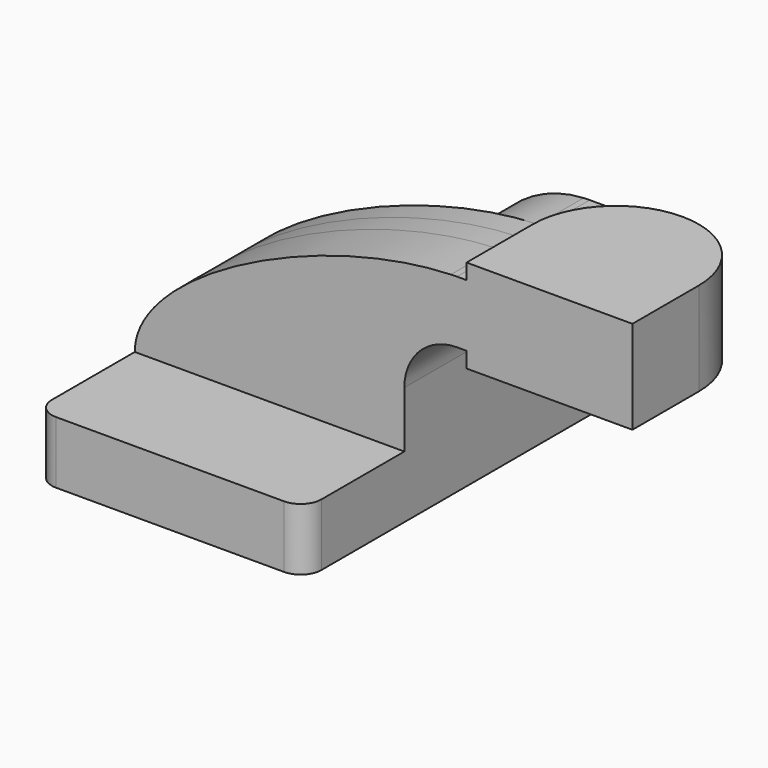
from build123d import *

# Parameters (mm, degrees)
F1_DEPTH = 63.5
F0_W     = 25.4
F0_H     = 19.05
F2_DEPTH = 25.4
F3_DEPTH = 7.9375
F5_R     = 6.35
F0_H_2   = 4.7752
F0_H_3   = 4.7498
F6_DEPTH = 25.4


with BuildPart() as f1:
    # F0 (on Front) → F1 (new body, symmetric)
    with BuildSketch(Plane.XZ):
        Polygon((-41.275, -9.525), (41.275, -9.525), (41.275, 9.525), (22.225, 9.525), (-41.275, 9.525), align=None)
    extrude(amount=F1_DEPTH, both=True)

    # F0 (on Front) → F2 (join, symmetric)
    with BuildSketch(Plane.XZ):
        with BuildLine():
            Line((22.225, 9.525), (41.275, 9.525))
            Line((41.275, 9.525), (41.275, 26.7462))
            ThreePointArc((41.275, 26.7462), (45.9990747262, 38.1511252738), (57.404, 42.8752))
            Line((57.404, 42.8752), (60.325, 42.8752))
            Line((60.325, 42.8752), (60.325, 61.9252))
            Line((60.325, 61.9252), (57.404, 61.9252))
            add(Edge.make_bspline(
                [(55.5422575952, 61.875901909), (56.1662788609, 61.89841175), (56.7869415526, 61.914880349), (57.404, 61.9252)],
                knots=[110.0591294768, 110.0591294768, 110.0591294768, 110.0591294768, 111.7288056011, 111.7288056011, 111.7288056011, 111.7288056011], degree=3))
            ThreePointArc((55.5422575952, 61.875901909), (31.8789507634, 50.9543371128), (22.225, 26.7462))
            Line((22.225, 26.7462), (22.225, 9.525))
        make_face()
        with Locations((73.025, 52.4002)):
            Rectangle(F0_W, F0_H)
    extrude(amount=F2_DEPTH, both=True)

    # F0 (on Front) → F3 (join, symmetric)
    with BuildSketch(Plane.XZ):
        with BuildLine():
            add(Edge.make_bspline(
                [(-41.275, 9.525), (-41.317213665, 32.6592953767), (14.4089885277, 60.3921330151), (55.5422575952, 61.875901909)],
                knots=[0, 0, 0, 0, 110.0591294768, 110.0591294768, 110.0591294768, 110.0591294768], degree=3))
            Line((-41.275, 9.525), (22.225, 9.525))
            Line((22.225, 9.525), (22.225, 26.7462))
            ThreePointArc((22.225, 26.7462), (31.8789507634, 50.9543371128), (55.5422575952, 61.875901909))
        make_face()
    extrude(amount=F3_DEPTH, both=True)

    # F0 (on Front) → F4 (revolve)
    with BuildSketch(Plane.XZ):
        Polygon((85.725, 61.9252), (85.725, 42.8752), (85.725, 38.1), (111.125, 38.1), (111.125, 66.675), (85.725, 66.675), align=None)
    revolve(axis=Axis((85.725, 0, 52.3875), (0, 0, -1)))

    # F5
    f5_edges = [f1.edges().sort_by_distance(p)[0] for p in [
        (-41.275, -63.5, 0),
        (41.275, -63.5, 0),
        (-41.275, 63.5, 0),
        (41.275, 63.5, 0),
    ]]
    fillet(f5_edges, radius=F5_R)

    # F0 (on Front) → F6 (join)
    with BuildSketch(Plane.XZ):
        Polygon((-41.275, -9.525), (41.275, -9.525), (41.275, 9.525), (22.225, 9.525), (-41.275, 9.525), align=None)
        with BuildLine():
            Line((22.225, 9.525), (41.275, 9.525))
            Line((41.275, 9.525), (41.275, 26.7462))
            ThreePointArc((41.275, 26.7462), (45.9990747262, 38.1511252738), (57.404, 42.8752))
            Line((57.404, 42.8752), (60.325, 42.8752))
            Line((60.325, 42.8752), (60.325, 61.9252))
            Line((60.325, 61.9252), (57.404, 61.9252))
            add(Edge.make_bspline(
                [(55.5422575952, 61.875901909), (56.1662788609, 61.89841175), (56.7869415526, 61.914880349), (57.404, 61.9252)],
                knots=[110.0591294768, 110.0591294768, 110.0591294768, 110.0591294768, 111.7288056011, 111.7288056011, 111.7288056011, 111.7288056011], degree=3))
            ThreePointArc((55.5422575952, 61.875901909), (31.8789507634, 50.9543371128), (22.225, 26.7462))
            Line((22.225, 26.7462), (22.225, 9.525))
        make_face()
        with BuildLine():
            add(Edge.make_bspline(
                [(-41.275, 9.525), (-41.317213665, 32.6592953767), (14.4089885277, 60.3921330151), (55.5422575952, 61.875901909)],
                knots=[0, 0, 0, 0, 110.0591294768, 110.0591294768, 110.0591294768, 110.0591294768], degree=3))
            Line((-41.275, 9.525), (22.225, 9.525))
            Line((22.225, 9.525), (22.225, 26.7462))
            ThreePointArc((22.225, 26.7462), (31.8789507634, 50.9543371128), (55.5422575952, 61.875901909))
        make_face()
        with Locations((73.025, 40.4876)):
            Rectangle(F0_W, F0_H_2)
        with Locations((73.025, 52.4002)):
            Rectangle(F0_W, F0_H)
        with Locations((73.025, 64.3001)):
            Rectangle(F0_W, F0_H_3)
        Polygon((85.725, 61.9252), (85.725, 42.8752), (85.725, 38.1), (111.125, 38.1), (111.125, 66.675), (85.725, 66.675), align=None)
    extrude(amount=F6_DEPTH)


solid = f1.part
